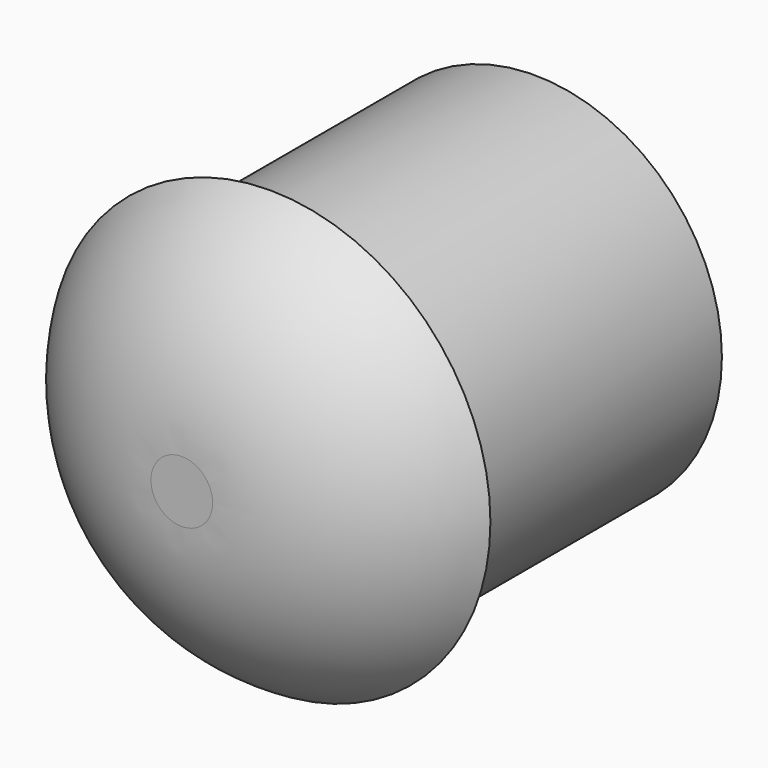
from build123d import *

# Parameters (mm, degrees)
F0_R     = 8.5
F1_DEPTH = 15
F2_R     = 10
F3_DEPTH = 5


# Not quite as in the source:
# - a fillet or chamfer that OpenCascade refuses, or shapes differently, is made with other operations: its cross-section is extruded or revolved along the edge and cut away or added


with BuildPart() as f1:
    # F0 (on Front) → F1 (new body)
    with BuildSketch(Plane.XZ):
        Circle(F0_R)
    extrude(amount=F1_DEPTH)

    # F2 (on face) → F3 (join)
    with BuildSketch(Plane.XZ.offset(15)):
        Circle(F2_R)
    extrude(amount=F3_DEPTH)

    # F4: fillet of radius 9.8982756057 on 1 edges, made by hand

    # F4_s1 → F4_t2 (revolve, cut)
    with BuildSketch(Plane.XY):
        with BuildLine():
            ThreePointArc((10, -15), (6.3731809715, -18.6591872749), (1.3986770752, -20))
            Line((1.3986770752, -20), (10, -20))
            Line((10, -20), (10, -15))
        make_face()
    revolve(axis=Axis((0, -20, 0), (0, -1, 0)), mode=Mode.SUBTRACT)


solid = f1.part
